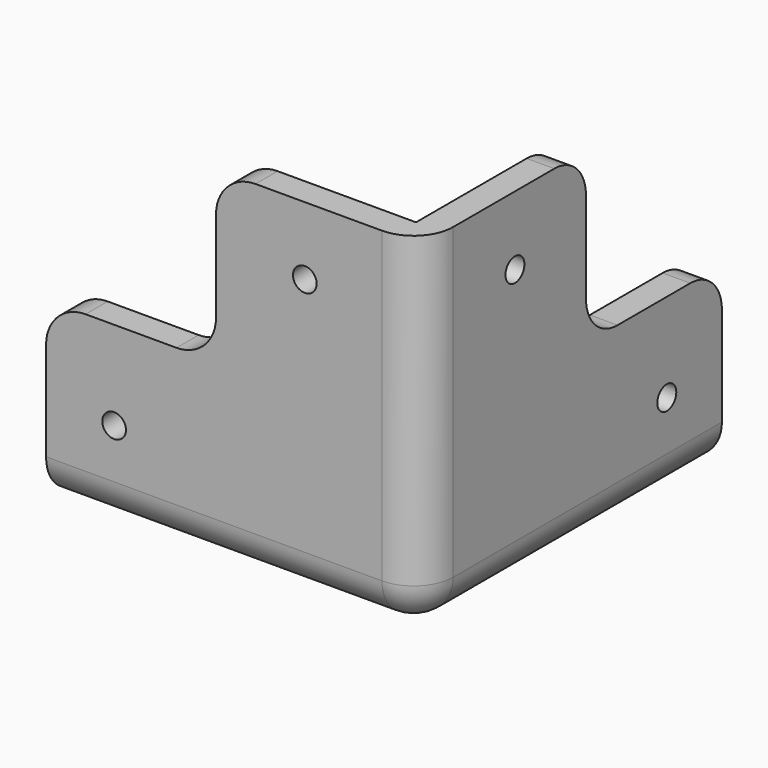
from build123d import *

# Parameters (mm, degrees)
F1_DEPTH  = 44
F2_T      = -3.5
F3_W      = 21.5
F3_H      = 21.5
F4_DEPTH  = 25
F5_W      = 21.5
F5_H      = 21.5
F6_DEPTH  = 25
F7_R      = 5
F10_R     = 1.5
F11_DEPTH = 25
F9_R      = 1.5
F12_DEPTH = 25
F8_R      = 1.5
F13_DEPTH = 25


with BuildPart() as f1:
    # F0 (on Top) → F1 (new body)
    with BuildSketch(Plane.XY):
        Polygon((0, 25), (0, 0), (-25, 0), (-25, -22.5), (0, -22.5), (22.5, -22.5), (22.5, 0), (22.5, 25), align=None)
    extrude(amount=F1_DEPTH)

    # F2
    f2_openings = [f1.faces().sort_by_distance(p)[0] for p in [
        (3.060345, -3.060345, 44),
        (0, 12.5, 22),
        (-12.5, 0, 22),
        (-25, -11.25, 22),
        (11.25, 25, 22),
    ]]
    offset(amount=F2_T, openings=f2_openings)

    # F3 (on face) → F4 (cut)
    with BuildSketch(Plane(origin=(19, 0, 0), x_dir=(0, -1, 0), z_dir=(-1, 0, 0))):
        with Locations((-14.25, 33.25)):
            Rectangle(F3_W, F3_H)
    extrude(amount=-F4_DEPTH, mode=Mode.SUBTRACT)

    # F5 (on face) → F6 (cut)
    with BuildSketch(Plane(origin=(0, -19, 0), x_dir=(-1, 0, 0), z_dir=(0, 1, 0))):
        with Locations((14.25, 33.25)):
            Rectangle(F5_W, F5_H)
    extrude(amount=-F6_DEPTH, mode=Mode.SUBTRACT)

    # F7
    f7_edges = [f1.edges().sort_by_distance(p)[0] for p in [
        (22.5, 1.25, 0),
        (-1.25, -22.5, 0),
        (22.5, -22.5, 22),
        (0, 0, 1.75),
        (-3.5, -20.75, 22.5),
        (0, 25, 1.75),
        (20.75, 25, 22.5),
        (-3.5, -20.75, 44),
        (-25, -20.75, 22.5),
        (-25, 0, 1.75),
        (20.75, 3.5, 22.5),
        (20.75, 3.5, 44),
    ]]
    fillet(f7_edges, radius=F7_R)

    # F10 (on face) → F11 (cut)
    with BuildSketch(Plane.XZ.offset(22.5)):
        with Locations((7.732233047, 35.3934139763)):
            Circle(F10_R)
        with Locations((-16.3934139763, 11.267766953)):
            Circle(F10_R)
    extrude(amount=-F11_DEPTH, mode=Mode.SUBTRACT)

    # F9 (on face) → F12 (cut)
    with BuildSketch(Plane.YZ.offset(22.5)):
        with Locations((-7.732233047, 35.2836836879)):
            Circle(F9_R)
        with Locations((16.2836836879, 11.267766953)):
            Circle(F9_R)
    extrude(amount=-F12_DEPTH, mode=Mode.SUBTRACT)

    # F8 (on face) → F13 (cut)
    with BuildSketch(Plane.XY.offset(3.5)):
        with Locations((-17.0746488054, -8.482233047)):
            Circle(F8_R)
        with Locations((8.482233047, 17.0746488054)):
            Circle(F8_R)
    extrude(amount=-F13_DEPTH, mode=Mode.SUBTRACT)


solid = f1.part
